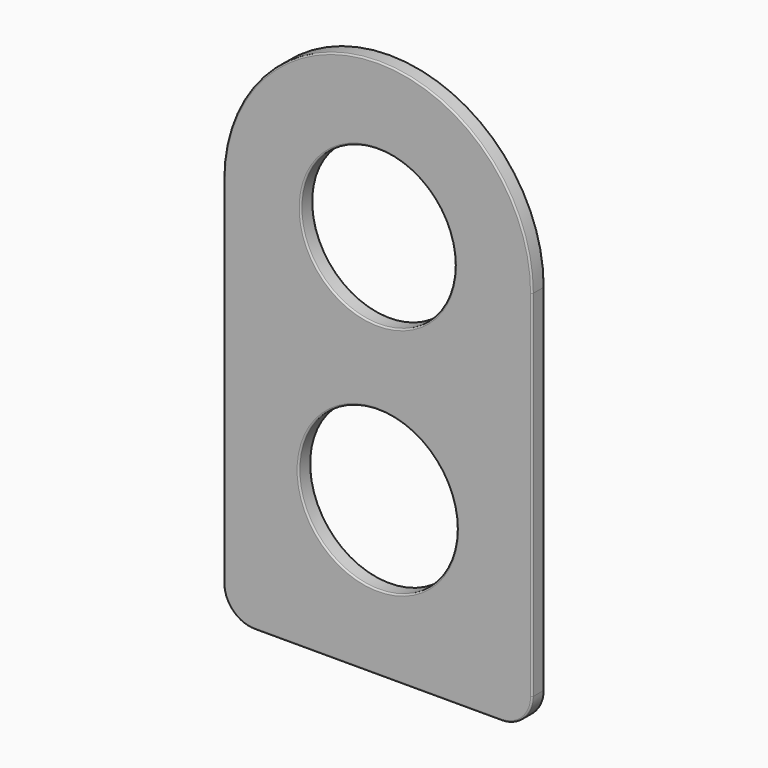
from build123d import *

# Parameters (mm, degrees)
F0_R     = 130.3580265026
F0_R_2   = 127
F1_DEPTH = 25.4
F2_R     = 2.54


# Not quite as in the source:
# - a feature names something its author has since deleted; it is built from what else it names


with BuildPart() as f1:
    # F0 (on Front) → F1 (new body)
    with BuildSketch(Plane.XZ):
        with BuildLine():
            ThreePointArc((-376.6236739159, -251.8737668991), (-361.7446984001, -287.7947913834), (-325.8236739159, -302.6737668991))
            Line((-325.8236739159, -302.6737668991), (80.5763260841, -302.6737668991))
            ThreePointArc((80.5763260841, -302.6737668991), (116.4973505684, -287.7947913834), (131.3763260841, -251.8737668991))
            Line((131.3763260841, -251.8737668991), (131.3763260841, 332.3262331009))
            ThreePointArc((131.3763260841, 332.3262331009), (56.9814485055, 511.9313555223), (-122.6236739159, 586.3262331009))
            ThreePointArc((-122.6236739159, 586.3262331009), (-302.2287963372, 511.9313555223), (-376.6236739159, 332.3262331009))
            Line((-376.6236739159, 332.3262331009), (-376.6236739159, -251.8737668991))
        make_face()
        with Locations((-122.6236739159, -48.6737668991)):
            Circle(F0_R, mode=Mode.SUBTRACT)
        with Locations((-122.6236739159, 332.3262331009)):
            Circle(F0_R_2, mode=Mode.SUBTRACT)
    extrude(amount=F1_DEPTH)

    # F2
    f2_edges = [f1.edges().sort_by_distance(p)[0] for p in [
        (131.376326, -25.4, 40.226233),
        (-122.623674, -25.4, -302.673767),
        (-376.623674, -25.4, 40.226233),
        (-122.623674, -25.4, 586.326233),
        (-249.623674, -25.4, 332.326233),
        (-249.623674, 0, 332.326233),
        (-376.623674, 0, 40.226233),
        (-122.623674, 0, 586.326233),
        (131.376326, 0, 40.226233),
        (-122.623674, 0, -302.673767),
        (-361.744698, 0, -287.794791),
        (116.497351, 0, -287.794791),
        (-252.9817, 0, -48.673767),
        (7.734353, -12.7, -48.673767),
        (-252.9817, -25.4, -48.673767),
        (-376.623674, -12.7, -251.873767),
        (-325.823674, -12.7, -302.673767),
        (-361.744698, -25.4, -287.794791),
        (116.497351, -25.4, -287.794791),
    ]]
    fillet(f2_edges, radius=F2_R)


solid = f1.part
